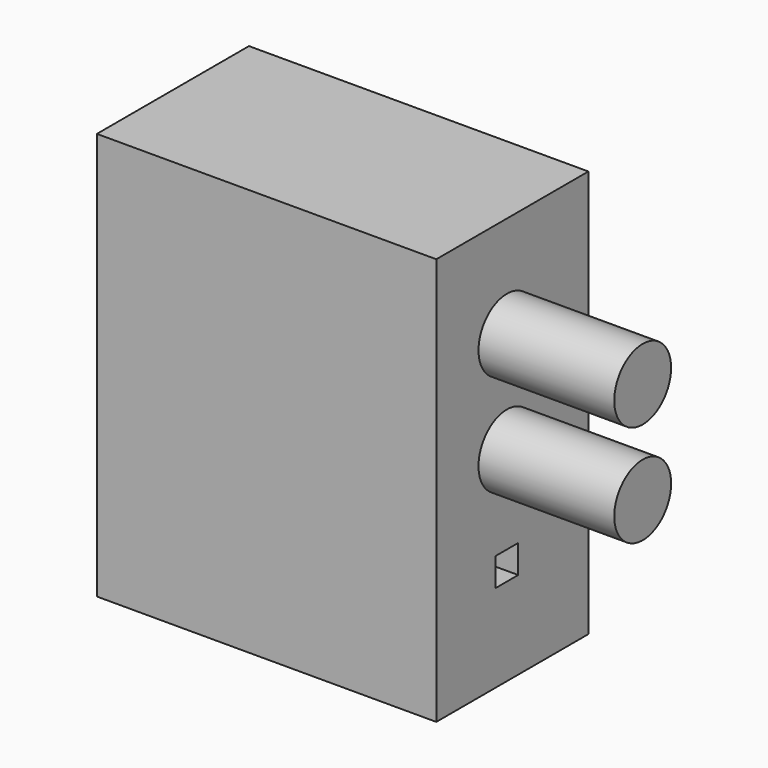
from build123d import *

# Parameters (mm, degrees)
F0_W     = 39.6875
F0_H     = 47.625
F1_DEPTH = 22.225
F2_R     = 4.1548957558
F3_DEPTH = 15.875
F2_W     = 3.302
F2_H     = 3.302
F4_DEPTH = 12.7


# Not quite as in the source:
# - a length typed as a fraction of an inch, garbled in the dataset ("3 / 203.2 mm" for 3/8 in), is restored


with BuildPart() as f1:
    # F0 (on Front) → F1 (new body)
    with BuildSketch(Plane.XZ):
        with Locations((-3.6287705289, -8.4221055731)):
            Rectangle(F0_W, F0_H)
    extrude(amount=F1_DEPTH)

    # F2 (on face) → F3 (join)
    with BuildSketch(Plane.YZ.offset(16.2149794711)):
        with Locations((-11.90625, 3.4968444269)):
            Circle(F2_R)
        with Locations((-11.90625, -8.4157555731)):
            Circle(F2_R)
    extrude(amount=F3_DEPTH)

    # F2 (on face) → F4 (cut)
    with BuildSketch(Plane.YZ.offset(16.2149794711)):
        with Locations((-11.90625, -20.3283555731)):
            Rectangle(F2_W, F2_H)
    extrude(amount=-F4_DEPTH, mode=Mode.SUBTRACT)


solid = f1.part
